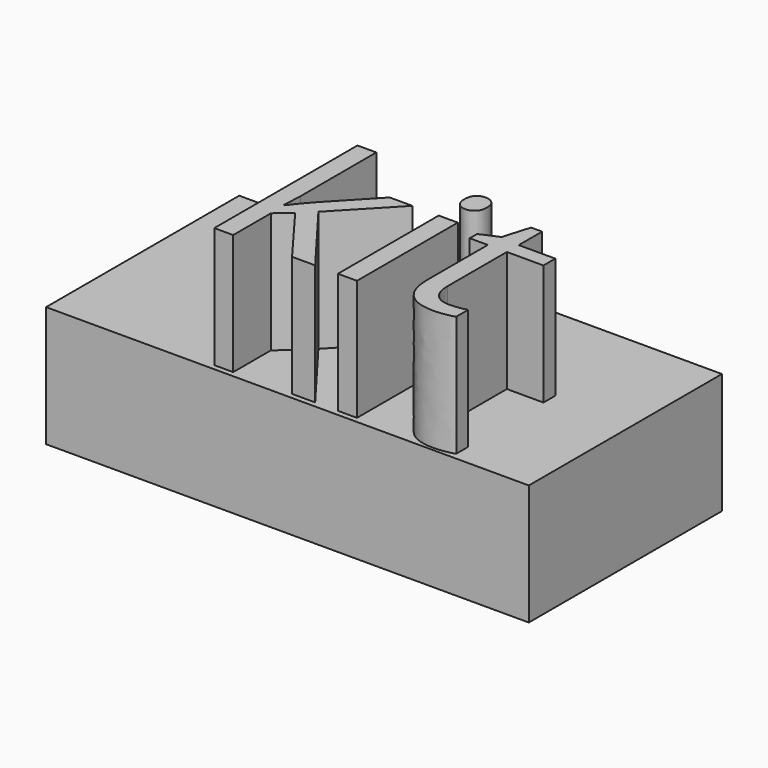
from build123d import *

# Parameters (mm, degrees)
F0_W         = 100
F0_H         = 50
F1_DEPTH     = 25
F3_TEXT_SIZE = 48.7780922817
F4_DEPTH     = 25


# Not quite as in the source:
# - Text() gives the source's letters only with a copy of the font that has no kerning and outlines rounded to 1/6400 em; it was checked with that copy


with BuildPart() as f1:
    # F0 (on Top) → F1 (new body)
    with BuildSketch(Plane.XY):
        with Locations((-6.4733318985, -11.2410843372)):
            Rectangle(F0_W, F0_H)
    extrude(amount=F1_DEPTH)


with BuildPart() as f4:
    # F3 (on offset) → F4 (new body, through all)
    with BuildSketch(Plane.XY.offset(50)):
        with Locations((-26.7137866467, -35.1202264428)):
            Text('kit', F3_TEXT_SIZE, font='Open Sans', text_align=(TextAlign.LEFT, TextAlign.BOTTOM))
    extrude(amount=-F4_DEPTH)


solid = Compound([f1.part, f4.part])
